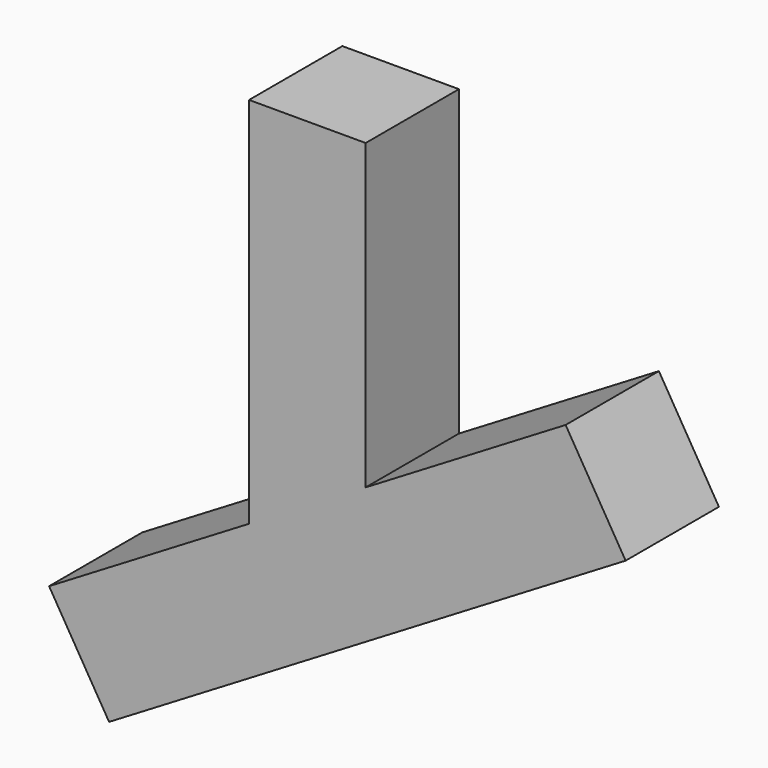
from build123d import *

# Parameters (mm, degrees)
F0_W            = 3.175
F0_H            = 10.16
F1_DEPTH        = 3.175
F2_SIZE2        = 3.17499
F2_SIZE         = 1.90499
F3_DEPTH        = 3.175
F4_DEPTH        = 6.35
F4_COPIES_COUNT = 2
F4_COPIES_PITCH = 10.052646


# Not quite as in the source:
# - a fillet or chamfer is up to 0.001 mm smaller than in the source, because OpenCascade refuses the exact size
# - a feature of the source that left no trace in its solid (it failed there, or was rolled back) is left out
# - a pattern or mirror of a feature is missing from the dataset's text; its kind, count and spacing are read off the source's solid


with BuildPart() as f1:
    # F0 (on Front) → F1 (new body)
    with BuildSketch(Plane.XZ):
        with Locations((1.5875, -5.08)):
            Rectangle(F0_W, F0_H)
    extrude(amount=F1_DEPTH)

    # F2 (size 1.905 and 3.175 in the source; OpenCascade refuses exactly that, so slightly less here)
    f2_edges = [f1.edges().sort_by_distance(p)[0] for p in [
        (3.175, -1.5875, -10.16),
    ]]
    f2_side = f1.faces().sort_by_distance((3.175, -1.5875, -5.08))[0]
    chamfer(f2_edges, length=F2_SIZE, length2=F2_SIZE2, reference=f2_side)


with BuildPart() as f3:
    # F3 (new): a face of the model
    f3_faces = [f1.part.faces().sort_by_distance(p)[0] for p in [
        (1.587505, -1.5875, -9.207505),
    ]]
    extrude(f3_faces, amount=F3_DEPTH)


with BuildPart() as f1_1:
    add(f1.part)

    # F4 (add): a face of the model
    f4_faces = [f3.part.faces().sort_by_distance(p)[0] for p in [
        (0.8167707507, -1.5875, -11.5212707762),
    ]]

    add(f3.part)  # F4 merges F3
    f4 = extrude(f4_faces, amount=F4_DEPTH)

    # F4_copies: F4 ×2
    with Locations(*[Vector(0.8574928129, 0, 0.5144959434) * (i * F4_COPIES_PITCH) for i in range(1, F4_COPIES_COUNT)]):
        add(f4)


solid = f1_1.part
